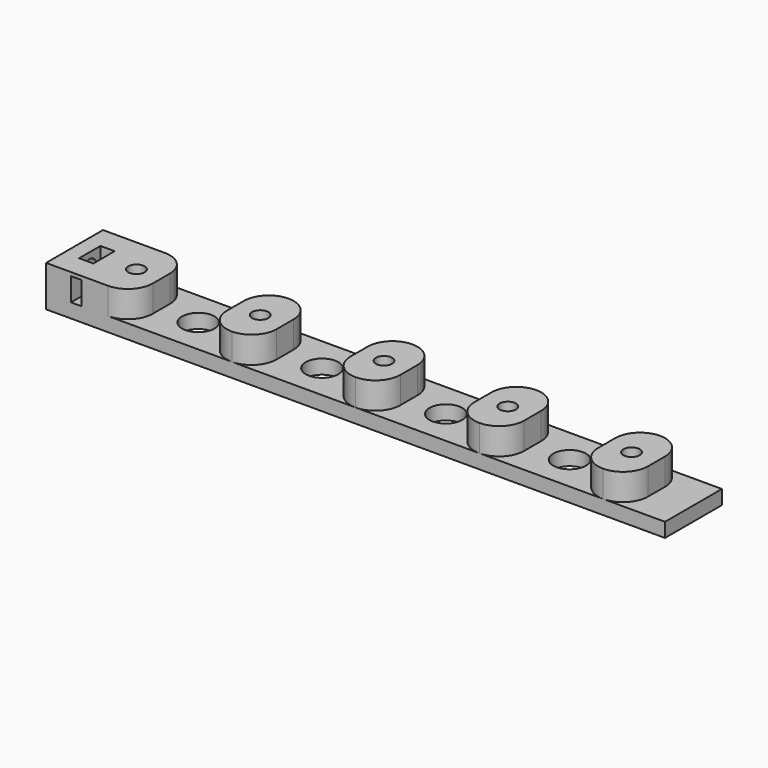
from build123d import *

# Parameters (mm, degrees)
F0_W           = 174
F0_H           = 20
F0_R           = 4.6
F1_DEPTH       = 4
F2_W           = 14
F2_H           = 20
F3_DEPTH       = 7.5
F5_D           = 4.6
F5_CBORE_D     = 7.5
F5_CBORE_DEPTH = 8
F6_R           = 6.99999
F7_DEPTH       = 7.5
F8_W           = 3
F8_H           = 6.5
F9_DEPTH       = 25
F10_W          = 4
F10_H          = 7.5
F11_DEPTH      = 7
F12_R          = 2.3
F13_DEPTH      = 10


# Not quite as in the source:
# - a fillet or chamfer is up to 0.001 mm smaller than in the source, because OpenCascade refuses the exact size


with BuildPart() as f1:
    # F0 (on Top) → F1 (new body)
    with BuildSketch(Plane.XY):
        with Locations((52.2, 0)):
            Rectangle(F0_W, F0_H)
        Circle(F0_R, mode=Mode.SUBTRACT)
        with Locations((34.8, 0)):
            Circle(F0_R, mode=Mode.SUBTRACT)
        with Locations((69.6, 0)):
            Circle(F0_R, mode=Mode.SUBTRACT)
        with Locations((104.4, 0)):
            Circle(F0_R, mode=Mode.SUBTRACT)
    extrude(amount=F1_DEPTH)

    # F2 (on face) → F3 (join)
    with BuildSketch(Plane.XY.offset(4)):
        with Locations((-17.4, 0)):
            Rectangle(F2_W, F2_H)
        with Locations((17.4, 0)):
            Rectangle(F2_W, F2_H)
        with Locations((52.2, 0)):
            Rectangle(F2_W, F2_H)
        with Locations((87, 0)):
            Rectangle(F2_W, F2_H)
        with Locations((121.8, 0)):
            Rectangle(F2_W, F2_H)
    extrude(amount=F3_DEPTH)

    # F5 (through all)
    with Locations(Plane(origin=(0, 0, 0), x_dir=(1, 0, 0), z_dir=(0, 0, -1))):
        with Locations((-17.4, 0), (17.4, 0), (52.2, 0), (87, 0), (121.8, 0)):
            CounterBoreHole(F5_D / 2, F5_CBORE_D / 2, F5_CBORE_DEPTH)

    # F6 (radius 7 in the source; OpenCascade refuses exactly that, so slightly less here)
    f6_edges = [f1.edges().sort_by_distance(p)[0] for p in [
        (-10.4, 10, 7.75),
        (10.4, 10, 7.75),
        (24.4, 10, 7.75),
        (45.2, 10, 7.75),
        (59.2, 10, 7.75),
        (80, 10, 7.75),
        (94, 10, 7.75),
        (128.8, 10, 7.75),
        (114.8, 10, 7.75),
        (-24.4, 10, 7.75),
        (-24.4, -10, 7.75),
        (-10.4, -10, 7.75),
        (10.4, -10, 7.75),
        (24.4, -10, 7.75),
        (45.2, -10, 7.75),
        (59.2, -10, 7.75),
        (80, -10, 7.75),
        (94, -10, 7.75),
        (114.8, -10, 7.75),
        (128.8, -10, 7.75),
    ]]
    fillet(f6_edges, radius=F6_R)

    # F7 (add): a face of the model
    f7_faces = [f1.faces().sort_by_distance(p)[0] for p in [
        (-28.9789302808, 0, 4),
    ]]
    extrude(f7_faces, amount=F7_DEPTH)

    # F8 (on face) → F9 (cut)
    with BuildSketch(Plane(origin=(0, 10, 0), x_dir=(-1, 0, 0), z_dir=(0, 1, 0))):
        with Locations((26.3, 7.25)):
            Rectangle(F8_W, F8_H)
    extrude(amount=-F9_DEPTH, mode=Mode.SUBTRACT)

    # F10 (on face) → F11 (cut)
    with BuildSketch(Plane.XY.offset(11.5)):
        with Locations((-28.5152019933, 0)):
            Rectangle(F10_W, F10_H)
    extrude(amount=-F11_DEPTH, mode=Mode.SUBTRACT)

    # F12 (on face) → F13 (cut)
    with BuildSketch(Plane(origin=(-34.8, 0, 0), x_dir=(0, -1, 0), z_dir=(-1, 0, 0))):
        with Locations((0, 7.5)):
            Circle(F12_R)
    extrude(amount=-F13_DEPTH, mode=Mode.SUBTRACT)


solid = f1.part
